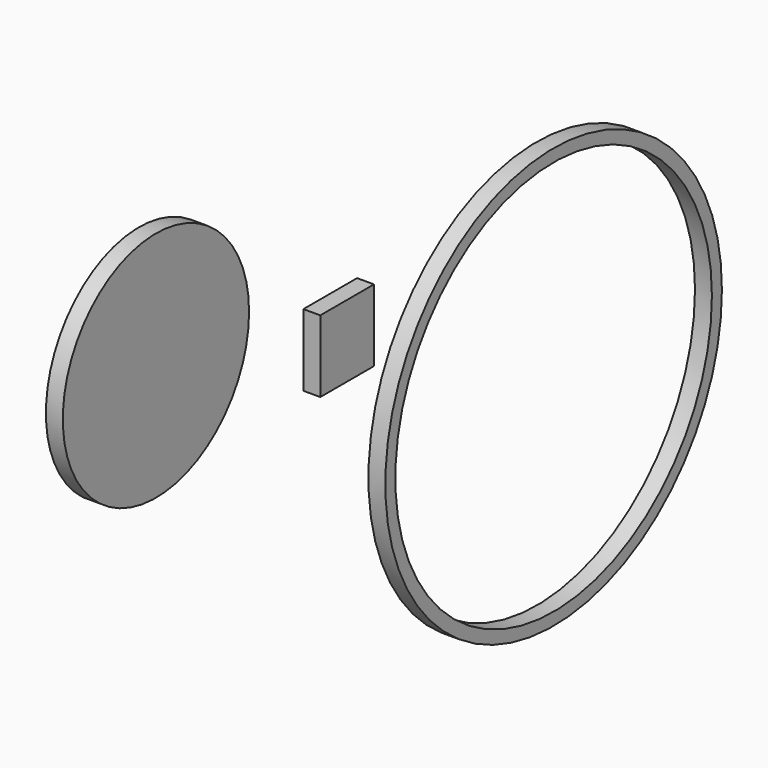
from build123d import *

# Parameters (mm, degrees)
F1_R     = 311
F1_R_2   = 292.5
F3_DEPTH = 25
F5_W     = 99.2197990417
F5_H     = 106.3870340586
F6_DEPTH = 25
F7_R     = 172.0890507053
F8_DEPTH = 25


# Not quite as in the source:
# - the program builds the solid bodies; features that only make, move or delete a surface that nothing else refers to are left out


with BuildPart() as f3:
    # F1 (on face) → F3 (new body)
    with BuildSketch(Plane.YZ):
        Circle(F1_R)
        Circle(F1_R_2, mode=Mode.SUBTRACT)
    extrude(amount=F3_DEPTH)


with BuildPart() as f6:
    # F5 (on Right) → F6 (new body)
    with BuildSketch(Plane.YZ):
        with Locations((-381.5611600876, 215.3727337718)):
            Rectangle(F5_W, F5_H)
    extrude(amount=F6_DEPTH)


with BuildPart() as f8:
    # F7 (on face) → F8 (new body)
    with BuildSketch(Plane.YZ.offset(25)):
        with Locations((-766.141474247, 347.4381864071)):
            Circle(F7_R)
    extrude(amount=F8_DEPTH)


solid = Compound([f3.part, f6.part, f8.part])
